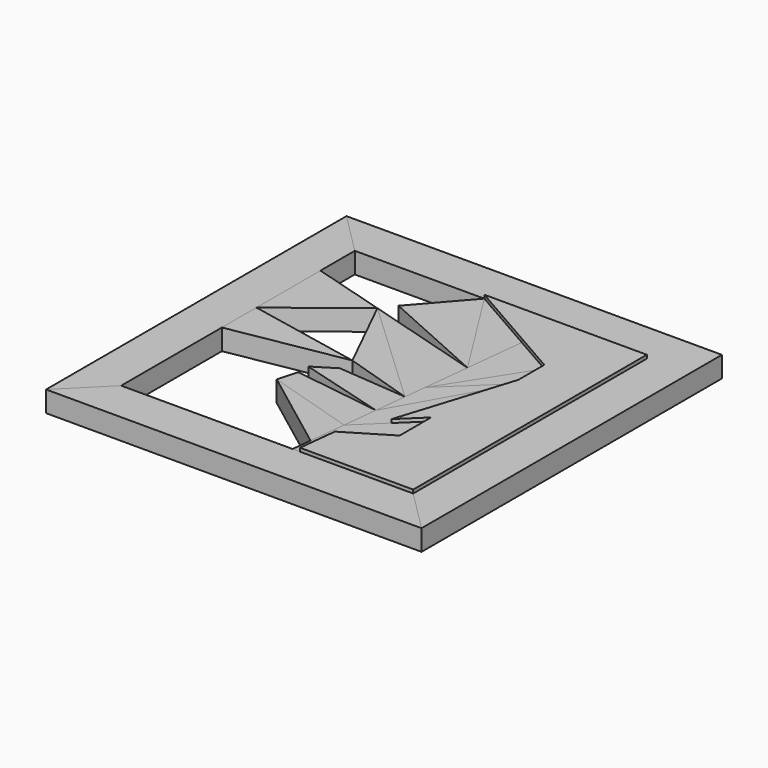
from build123d import *

# Parameters (mm, degrees)
F1_DEPTH  = 9.525
F2_DEPTH  = 9.525
F3_DEPTH  = 9.525
F4_DEPTH  = 9.525
F5_DEPTH  = 9.525
F6_DEPTH  = 9.525
F7_DEPTH  = 9.525
F8_DEPTH  = 9.525
F9_DEPTH  = 9.525
F10_DEPTH = 9.525
F11_DEPTH = 9.525
F12_DEPTH = 9.525
F13_DEPTH = 9.525
F14_DEPTH = 9.525
F15_DEPTH = 9.525
F16_DEPTH = 9.525
F17_DEPTH = 9.525
F18_DEPTH = 9.525
F19_DEPTH = 9.525
F20_DEPTH = 12.7


with BuildPart() as f1:
    # F0 (on Top) → F1 (new body, symmetric)
    with BuildSketch(Plane.XY):
        Polygon((-171.45, 171.45), (-171.45, -171.45), (-133.35, -133.35), (-133.35, -18.3831825852), (-133.35, 21.0410188884), (-133.35, 94.1308289766), (-133.35, 133.35), align=None)
    extrude(amount=F1_DEPTH, both=True)


with BuildPart() as f2:
    # F0 (on Top) → F2 (new body, symmetric)
    with BuildSketch(Plane.XY):
        Polygon((171.45, 171.45), (-171.45, 171.45), (-133.35, 133.35), (-85.5590856828, 133.35), (-15.077165328, 133.35), (133.35, 133.35), align=None)
    extrude(amount=F2_DEPTH, both=True)

    # F0 (on Top) → F3 (join, symmetric)
    with BuildSketch(Plane.XY):
        Polygon((133.35, -133.35), (171.45, -171.45), (171.45, 171.45), (133.35, 133.35), align=None)
    extrude(amount=F3_DEPTH, both=True)


with BuildPart() as f4:
    # F0 (on Top) → F4 (new body, symmetric)
    with BuildSketch(Plane.XY):
        Polygon((-133.35, -133.35), (-171.45, -171.45), (171.45, -171.45), (133.35, -133.35), (29.9828406423, -133.35), (23.2006912545, -133.35), align=None)
    extrude(amount=F4_DEPTH, both=True)


with BuildPart() as f5:
    # F0 (on Top) → F5 (new body, symmetric)
    with BuildSketch(Plane.XY):
        Polygon((42.2602014288, 42.4880021912), (-15.077165328, 133.35), (-56.0195036232, 86.5388959646), align=None)
    extrude(amount=F5_DEPTH, both=True)


with BuildPart() as f6:
    # F0 (on Top) → F6 (new body, symmetric)
    with BuildSketch(Plane.XY):
        Polygon((-52.7975902858, -56.4470457543), (25.1575205185, -115.2968105278), (26.521067056, -102.7170906481), (28.8153099508, -81.5510122196), align=None)
    extrude(amount=F6_DEPTH, both=True)


with BuildPart() as f7:
    # F0 (on Top) → F7 (new body, symmetric)
    with BuildSketch(Plane.XY):
        Polygon((26.521067056, -102.7170906481), (33.8283727055, -98.3124413095), (73.7134516239, -74.2707774043), (73.7134516239, -38.3952504957), (53.3703944978, -57.9488465546), (28.8153099508, -81.5510122196), align=None)
    extrude(amount=F7_DEPTH, both=True)


with BuildPart() as f8:
    # F0 (on Top) → F8 (new body, symmetric)
    with BuildSketch(Plane.XY):
        Polygon((86.0454812646, 45.9258191538), (32.2778299451, -49.606718123), (28.8153099508, -81.5510122196), (53.3703944978, -57.9488465546), align=None)
    extrude(amount=F8_DEPTH, both=True)


with BuildPart() as f9:
    # F0 (on Top) → F9 (new body, symmetric)
    with BuildSketch(Plane.XY):
        Polygon((28.8153099508, -81.5510122196), (32.2778299451, -49.606718123), (-47.6337224245, -38.2612505928), (-52.7975902858, -56.4470457543), align=None)
    extrude(amount=F9_DEPTH, both=True)


with BuildPart() as f10:
    # F0 (on Top) → F10 (new body, symmetric)
    with BuildSketch(Plane.XY):
        Polygon((32.2778299451, -49.606718123), (-28.3199971136, -14.9760207202), (-47.6337224245, -26.9157830626), align=None)
    extrude(amount=F10_DEPTH, both=True)

    # F0 (on Top) → F11 (join, symmetric)
    with BuildSketch(Plane.XY):
        Polygon((35.4441672467, -20.3949272483), (-28.3199971136, -14.9760207202), (32.2778299451, -49.606718123), align=None)
    extrude(amount=F11_DEPTH, both=True)


with BuildPart() as f12:
    # F0 (on Top) → F12 (new body, symmetric)
    with BuildSketch(Plane.XY):
        Polygon((37.6548231832, 0), (35.4441672467, -20.3949272483), (32.2778299451, -49.606718123), (86.0454812646, 45.9258191538), align=None)
    extrude(amount=F12_DEPTH, both=True)


with BuildPart() as f13:
    # F0 (on Top) → F13 (new body, symmetric)
    with BuildSketch(Plane.XY):
        Polygon((86.0454812646, 75.4573446445), (37.6548231832, 0), (86.0454812646, 45.9258191538), align=None)
    extrude(amount=F13_DEPTH, both=True)


with BuildPart() as f14:
    # F0 (on Top) → F14 (new body, symmetric)
    with BuildSketch(Plane.XY):
        Polygon((86.0454812646, 75.4573446445), (48.1833487104, 97.1333931346), (42.2602014288, 42.4880021912), (37.6548231832, 0), align=None)
    extrude(amount=F14_DEPTH, both=True)


with BuildPart() as f15:
    # F0 (on Top) → F15 (new body, symmetric)
    with BuildSketch(Plane.XY):
        Polygon((48.1833487104, 97.1333931346), (-15.077165328, 133.35), (42.2602014288, 42.4880021912), align=None)
    extrude(amount=F15_DEPTH, both=True)


with BuildPart() as f16:
    # F0 (on Top) → F16 (new body, symmetric)
    with BuildSketch(Plane.XY):
        Polygon((42.2602014288, 42.4880021912), (-65.3918460011, 74.2068663239), (35.4441672467, -20.3949272483), (37.6548231832, 0), align=None)
    extrude(amount=F16_DEPTH, both=True)


with BuildPart() as f17:
    # F0 (on Top) → F17 (new body, symmetric)
    with BuildSketch(Plane.XY):
        Polygon((-65.3918460011, 74.2068663239), (-28.8890395314, 0), (35.4441672467, -20.3949272483), align=None)
    extrude(amount=F17_DEPTH, both=True)


with BuildPart() as f18:
    # F0 (on Top) → F18 (new body, symmetric)
    with BuildSketch(Plane.XY):
        Polygon((25.1575205185, -115.2968105278), (23.2006912545, -133.35), (29.9828406423, -133.35), (33.8283727055, -98.3124413095), (26.521067056, -102.7170906481), align=None)
    extrude(amount=F18_DEPTH, both=True)


with BuildPart() as f19:
    # F0 (on Top) → F19 (new body, symmetric)
    with BuildSketch(Plane.XY):
        Polygon((-133.35, 21.0410188884), (-133.35, -18.3831825852), (-28.8890395314, 0), align=None)
    extrude(amount=F19_DEPTH, both=True)


with BuildPart() as f19b:
    # F0 (on Top) → F19, piece 2 (new body, symmetric)
    with BuildSketch(Plane.XY):
        Polygon((-65.3918460011, 74.2068663239), (-133.35, 94.1308289766), (-133.35, 21.0410188884), align=None)
    extrude(amount=F19_DEPTH, both=True)


with BuildPart() as f20:
    # F0 (on Top) → F20 (new body, symmetric)
    with BuildSketch(Plane.XY):
        Polygon((29.9828406423, -133.35), (133.35, -133.35), (133.35, 133.35), (-15.077165328, 133.35), (48.1833487104, 97.1333931346), (86.0454812646, 75.4573446445), (86.0454812646, 45.9258191538), (53.3703944978, -57.9488465546), (73.7134516239, -38.3952504957), (73.7134516239, -74.2707774043), (33.8283727055, -98.3124413095), align=None)
    extrude(amount=F20_DEPTH, both=True)


solid = Compound([f1.part, f2.part, f4.part, f5.part, f6.part, f7.part, f8.part, f9.part, f10.part, f12.part, f13.part, f14.part, f15.part, f16.part, f17.part, f18.part, f19.part, f19b.part, f20.part])
